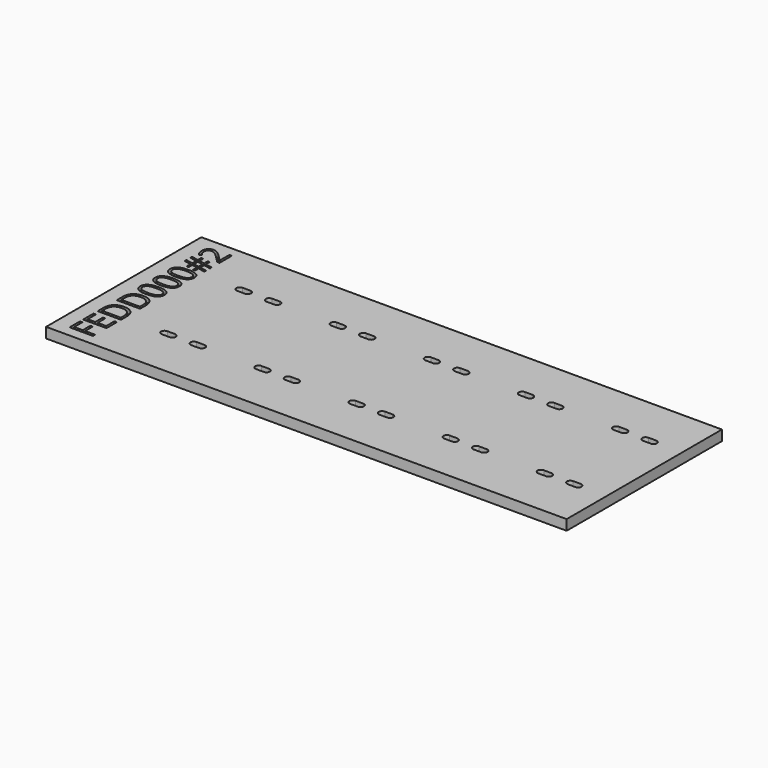
from build123d import *

# Parameters (mm, degrees)
F0_W         = 177
F0_H         = 66
F1_DEPTH     = 3.5
F2_TEXT_SIZE = 11.1111111111
F3_DEPTH     = 1.5
F5_DEPTH     = 3.5
F6_T1_DEPTH  = 3.5


# Not quite as in the source:
# - a fillet or chamfer that OpenCascade refuses, or shapes differently, is made with other operations: its cross-section is extruded or revolved along the edge and cut away or added
# - Text() gives the source's letters only with a copy of the font that has no kerning and outlines rounded to 1/6400 em; it was checked with that copy


with BuildPart() as f1:
    # F0 (on Top) → F1 (new body)
    with BuildSketch(Plane.XY):
        with Locations((0.9526101351, -16.284535466)):
            Rectangle(F0_W, F0_H)
    extrude(amount=F1_DEPTH)

    # F2 (on face) → F3 (cut)
    with BuildSketch(Plane.XY.offset(3.5)):
        with Locations(Location((-74.5473898649, -46.697535466), (0, 0, 90))):
            Text('FEDD000#2', F2_TEXT_SIZE, font='Open Sans', text_align=(TextAlign.LEFT, TextAlign.BOTTOM))
    extrude(amount=-F3_DEPTH, mode=Mode.SUBTRACT)

    # F4 (on face) → F5 (cut, through all)
    with BuildSketch(Plane.XY.offset(3.5)):
        with BuildLine():
            ThreePointArc((-59.5473898649, -1.434535466), (-58.7342170666, -1.0977082644), (-58.3973898649, -0.284535466))
            ThreePointArc((-58.3973898649, -0.284535466), (-58.7342170666, 0.5286373324), (-59.5473898649, 0.865464534))
            ThreePointArc((-59.5473898649, 0.865464534), (-60.6973898649, -0.284535466), (-59.5473898649, -1.434535466))
        make_face()
        with BuildLine():
            ThreePointArc((-59.5473898649, 0.865464534), (-58.7342170666, 0.5286373324), (-58.3973898649, -0.284535466))
            ThreePointArc((-58.3973898649, -0.284535466), (-58.7342170666, -1.0977082644), (-59.5473898649, -1.434535466))
            Line((-59.5473898649, -1.434535466), (-57.0473898649, -1.434535466))
            Line((-57.0473898649, -1.434535466), (-57.0473898649, 0.865464534))
            Line((-57.0473898649, 0.865464534), (-59.5473898649, 0.865464534))
        make_face()
        with BuildLine():
            ThreePointArc((-59.5473898649, -1.434535466), (-60.6973898649, -0.284535466), (-59.5473898649, 0.865464534))
            Line((-59.5473898649, 0.865464534), (-62.0473898649, 0.865464534))
            Line((-62.0473898649, 0.865464534), (-62.0473898649, -1.434535466))
            Line((-62.0473898649, -1.434535466), (-59.5473898649, -1.434535466))
        make_face()
        with BuildLine():
            ThreePointArc((-49.5473898649, -1.434535466), (-48.7342170666, -1.0977082644), (-48.3973898649, -0.284535466))
            ThreePointArc((-48.3973898649, -0.284535466), (-48.7342170666, 0.5286373324), (-49.5473898649, 0.865464534))
            ThreePointArc((-49.5473898649, 0.865464534), (-50.6973898649, -0.284535466), (-49.5473898649, -1.434535466))
        make_face()
        with BuildLine():
            ThreePointArc((-49.5473898649, 0.865464534), (-48.7342170666, 0.5286373324), (-48.3973898649, -0.284535466))
            ThreePointArc((-48.3973898649, -0.284535466), (-48.7342170666, -1.0977082644), (-49.5473898649, -1.434535466))
            Line((-49.5473898649, -1.434535466), (-47.0473898649, -1.434535466))
            Line((-47.0473898649, -1.434535466), (-47.0473898649, 0.865464534))
            Line((-47.0473898649, 0.865464534), (-49.5473898649, 0.865464534))
        make_face()
        with BuildLine():
            ThreePointArc((-49.5473898649, -1.434535466), (-50.6973898649, -0.284535466), (-49.5473898649, 0.865464534))
            Line((-49.5473898649, 0.865464534), (-52.0473898649, 0.865464534))
            Line((-52.0473898649, 0.865464534), (-52.0473898649, -1.434535466))
            Line((-52.0473898649, -1.434535466), (-49.5473898649, -1.434535466))
        make_face()
        with BuildLine():
            ThreePointArc((-27.5473898649, -1.434535466), (-26.7342170666, -1.0977082644), (-26.3973898649, -0.284535466))
            ThreePointArc((-26.3973898649, -0.284535466), (-26.7342170666, 0.5286373324), (-27.5473898649, 0.865464534))
            ThreePointArc((-27.5473898649, 0.865464534), (-28.6973898649, -0.284535466), (-27.5473898649, -1.434535466))
        make_face()
        with BuildLine():
            ThreePointArc((-27.5473898649, 0.865464534), (-26.7342170666, 0.5286373324), (-26.3973898649, -0.284535466))
            ThreePointArc((-26.3973898649, -0.284535466), (-26.7342170666, -1.0977082644), (-27.5473898649, -1.434535466))
            Line((-27.5473898649, -1.434535466), (-25.0473898649, -1.434535466))
            Line((-25.0473898649, -1.434535466), (-25.0473898649, 0.865464534))
            Line((-25.0473898649, 0.865464534), (-27.5473898649, 0.865464534))
        make_face()
        with BuildLine():
            ThreePointArc((-27.5473898649, -1.434535466), (-28.6973898649, -0.284535466), (-27.5473898649, 0.865464534))
            Line((-27.5473898649, 0.865464534), (-30.0473898649, 0.865464534))
            Line((-30.0473898649, 0.865464534), (-30.0473898649, -1.434535466))
            Line((-30.0473898649, -1.434535466), (-27.5473898649, -1.434535466))
        make_face()
        with BuildLine():
            ThreePointArc((-17.5473898649, -1.434535466), (-16.7342170666, -1.0977082644), (-16.3973898649, -0.284535466))
            ThreePointArc((-16.3973898649, -0.284535466), (-16.7342170666, 0.5286373324), (-17.5473898649, 0.865464534))
            ThreePointArc((-17.5473898649, 0.865464534), (-18.6973898649, -0.284535466), (-17.5473898649, -1.434535466))
        make_face()
        with BuildLine():
            ThreePointArc((-17.5473898649, 0.865464534), (-16.7342170666, 0.5286373324), (-16.3973898649, -0.284535466))
            ThreePointArc((-16.3973898649, -0.284535466), (-16.7342170666, -1.0977082644), (-17.5473898649, -1.434535466))
            Line((-17.5473898649, -1.434535466), (-15.0473898649, -1.434535466))
            Line((-15.0473898649, -1.434535466), (-15.0473898649, 0.865464534))
            Line((-15.0473898649, 0.865464534), (-17.5473898649, 0.865464534))
        make_face()
        with BuildLine():
            ThreePointArc((-17.5473898649, -1.434535466), (-18.6973898649, -0.284535466), (-17.5473898649, 0.865464534))
            Line((-17.5473898649, 0.865464534), (-20.0473898649, 0.865464534))
            Line((-20.0473898649, 0.865464534), (-20.0473898649, -1.434535466))
            Line((-20.0473898649, -1.434535466), (-17.5473898649, -1.434535466))
        make_face()
        with BuildLine():
            ThreePointArc((4.4526101351, -1.434535466), (5.2657829334, -1.0977082644), (5.6026101351, -0.284535466))
            ThreePointArc((5.6026101351, -0.284535466), (5.2657829334, 0.5286373324), (4.4526101351, 0.865464534))
            ThreePointArc((4.4526101351, 0.865464534), (3.3026101351, -0.284535466), (4.4526101351, -1.434535466))
        make_face()
        with BuildLine():
            ThreePointArc((4.4526101351, 0.865464534), (5.2657829334, 0.5286373324), (5.6026101351, -0.284535466))
            ThreePointArc((5.6026101351, -0.284535466), (5.2657829334, -1.0977082644), (4.4526101351, -1.434535466))
            Line((4.4526101351, -1.434535466), (6.9526101351, -1.434535466))
            Line((6.9526101351, -1.434535466), (6.9526101351, 0.865464534))
            Line((6.9526101351, 0.865464534), (4.4526101351, 0.865464534))
        make_face()
        with BuildLine():
            ThreePointArc((4.4526101351, -1.434535466), (3.3026101351, -0.284535466), (4.4526101351, 0.865464534))
            Line((4.4526101351, 0.865464534), (1.9526101351, 0.865464534))
            Line((1.9526101351, 0.865464534), (1.9526101351, -1.434535466))
            Line((1.9526101351, -1.434535466), (4.4526101351, -1.434535466))
        make_face()
        with BuildLine():
            ThreePointArc((14.4526101316, -1.434535466), (15.2657829322, -1.0977082656), (15.6026101351, -0.284535466))
            ThreePointArc((15.6026101351, -0.284535466), (15.2657829334, 0.5286373324), (14.4526101351, 0.865464534))
            ThreePointArc((14.4526101351, 0.865464534), (13.3026101351, -0.2845354643), (14.4526101316, -1.434535466))
        make_face()
        with BuildLine():
            ThreePointArc((14.4526101351, 0.865464534), (15.2657829334, 0.5286373324), (15.6026101351, -0.284535466))
            ThreePointArc((15.6026101351, -0.284535466), (15.2657829322, -1.0977082656), (14.4526101316, -1.434535466))
            Line((14.4526101316, -1.434535466), (16.9526101351, -1.434535466))
            Line((16.9526101351, -1.434535466), (16.9526101351, 0.865464534))
            Line((16.9526101351, 0.865464534), (14.4526101351, 0.865464534))
        make_face()
        with BuildLine():
            ThreePointArc((14.4526101316, -1.434535466), (13.3026101351, -0.2845354643), (14.4526101351, 0.865464534))
            Line((14.4526101351, 0.865464534), (11.9526101351, 0.865464534))
            Line((11.9526101351, 0.865464534), (11.9526101351, -1.434535466))
            Line((11.9526101351, -1.434535466), (14.4526101316, -1.434535466))
        make_face()
        with BuildLine():
            ThreePointArc((36.4526101351, -1.434535466), (37.2657829334, -1.0977082644), (37.6026101351, -0.284535466))
            ThreePointArc((37.6026101351, -0.284535466), (37.2657829334, 0.5286373324), (36.4526101351, 0.865464534))
            ThreePointArc((36.4526101351, 0.865464534), (35.3026101351, -0.284535466), (36.4526101351, -1.434535466))
        make_face()
        with BuildLine():
            ThreePointArc((36.4526101351, 0.865464534), (37.2657829334, 0.5286373324), (37.6026101351, -0.284535466))
            ThreePointArc((37.6026101351, -0.284535466), (37.2657829334, -1.0977082644), (36.4526101351, -1.434535466))
            Line((36.4526101351, -1.434535466), (38.9526101351, -1.434535466))
            Line((38.9526101351, -1.434535466), (38.9526101351, 0.865464534))
            Line((38.9526101351, 0.865464534), (36.4526101351, 0.865464534))
        make_face()
        with BuildLine():
            ThreePointArc((36.4526101351, -1.434535466), (35.3026101351, -0.284535466), (36.4526101351, 0.865464534))
            Line((36.4526101351, 0.865464534), (33.9526101351, 0.865464534))
            Line((33.9526101351, 0.865464534), (33.9526101351, -1.434535466))
            Line((33.9526101351, -1.434535466), (36.4526101351, -1.434535466))
        make_face()
        with BuildLine():
            ThreePointArc((46.4526101351, -1.434535466), (47.2657829334, -1.0977082644), (47.6026101351, -0.284535466))
            ThreePointArc((47.6026101351, -0.284535466), (47.2657829334, 0.5286373324), (46.4526101351, 0.865464534))
            ThreePointArc((46.4526101351, 0.865464534), (45.3026101351, -0.284535466), (46.4526101351, -1.434535466))
        make_face()
        with BuildLine():
            ThreePointArc((46.4526101351, 0.865464534), (47.2657829334, 0.5286373324), (47.6026101351, -0.284535466))
            ThreePointArc((47.6026101351, -0.284535466), (47.2657829334, -1.0977082644), (46.4526101351, -1.434535466))
            Line((46.4526101351, -1.434535466), (48.9526101351, -1.434535466))
            Line((48.9526101351, -1.434535466), (48.9526101351, 0.865464534))
            Line((48.9526101351, 0.865464534), (46.4526101351, 0.865464534))
        make_face()
        with BuildLine():
            ThreePointArc((46.4526101351, -1.434535466), (45.3026101351, -0.284535466), (46.4526101351, 0.865464534))
            Line((46.4526101351, 0.865464534), (43.9526101351, 0.865464534))
            Line((43.9526101351, 0.865464534), (43.9526101351, -1.434535466))
            Line((43.9526101351, -1.434535466), (46.4526101351, -1.434535466))
        make_face()
        with BuildLine():
            ThreePointArc((68.4526101316, -1.434535466), (69.2657829322, -1.0977082656), (69.6026101351, -0.284535466))
            ThreePointArc((69.6026101351, -0.284535466), (69.2657829334, 0.5286373324), (68.4526101351, 0.865464534))
            ThreePointArc((68.4526101351, 0.865464534), (67.3026101351, -0.2845354643), (68.4526101316, -1.434535466))
        make_face()
        with BuildLine():
            ThreePointArc((68.4526101351, 0.865464534), (69.2657829334, 0.5286373324), (69.6026101351, -0.284535466))
            ThreePointArc((69.6026101351, -0.284535466), (69.2657829322, -1.0977082656), (68.4526101316, -1.434535466))
            Line((68.4526101316, -1.434535466), (70.9526101351, -1.434535466))
            Line((70.9526101351, -1.434535466), (70.9526101351, 0.865464534))
            Line((70.9526101351, 0.865464534), (68.4526101351, 0.865464534))
        make_face()
        with BuildLine():
            ThreePointArc((68.4526101316, -1.434535466), (67.3026101351, -0.2845354643), (68.4526101351, 0.865464534))
            Line((68.4526101351, 0.865464534), (65.9526101351, 0.865464534))
            Line((65.9526101351, 0.865464534), (65.9526101351, -1.434535466))
            Line((65.9526101351, -1.434535466), (68.4526101316, -1.434535466))
        make_face()
        with BuildLine():
            ThreePointArc((78.4526101351, -1.434535466), (79.2657829334, -1.0977082644), (79.6026101351, -0.284535466))
            ThreePointArc((79.6026101351, -0.284535466), (79.2657829334, 0.5286373324), (78.4526101351, 0.865464534))
            ThreePointArc((78.4526101351, 0.865464534), (77.3026101351, -0.284535466), (78.4526101351, -1.434535466))
        make_face()
        with BuildLine():
            ThreePointArc((78.4526101351, 0.865464534), (79.2657829334, 0.5286373324), (79.6026101351, -0.284535466))
            ThreePointArc((79.6026101351, -0.284535466), (79.2657829334, -1.0977082644), (78.4526101351, -1.434535466))
            Line((78.4526101351, -1.434535466), (80.9526101351, -1.434535466))
            Line((80.9526101351, -1.434535466), (80.9526101351, 0.865464534))
            Line((80.9526101351, 0.865464534), (78.4526101351, 0.865464534))
        make_face()
        with BuildLine():
            ThreePointArc((78.4526101351, -1.434535466), (77.3026101351, -0.284535466), (78.4526101351, 0.865464534))
            Line((78.4526101351, 0.865464534), (75.9526101351, 0.865464534))
            Line((75.9526101351, 0.865464534), (75.9526101351, -1.434535466))
            Line((75.9526101351, -1.434535466), (78.4526101351, -1.434535466))
        make_face()
        with BuildLine():
            ThreePointArc((-59.5473898649, -33.434535466), (-58.7342170666, -33.0977082644), (-58.3973898649, -32.284535466))
            ThreePointArc((-58.3973898649, -32.284535466), (-58.7342170666, -31.4713626676), (-59.5473898649, -31.134535466))
            ThreePointArc((-59.5473898649, -31.134535466), (-60.6973898649, -32.284535466), (-59.5473898649, -33.434535466))
        make_face()
        with BuildLine():
            ThreePointArc((-59.5473898649, -31.134535466), (-58.7342170666, -31.4713626676), (-58.3973898649, -32.284535466))
            ThreePointArc((-58.3973898649, -32.284535466), (-58.7342170666, -33.0977082644), (-59.5473898649, -33.434535466))
            Line((-59.5473898649, -33.434535466), (-57.0473898649, -33.434535466))
            Line((-57.0473898649, -33.434535466), (-57.0473898649, -31.134535466))
            Line((-57.0473898649, -31.134535466), (-59.5473898649, -31.134535466))
        make_face()
        with BuildLine():
            ThreePointArc((-59.5473898649, -33.434535466), (-60.6973898649, -32.284535466), (-59.5473898649, -31.134535466))
            Line((-59.5473898649, -31.134535466), (-62.0473898649, -31.134535466))
            Line((-62.0473898649, -31.134535466), (-62.0473898649, -33.434535466))
            Line((-62.0473898649, -33.434535466), (-59.5473898649, -33.434535466))
        make_face()
        with BuildLine():
            ThreePointArc((-49.5473898649, -33.434535466), (-48.7342170666, -33.0977082644), (-48.3973898649, -32.284535466))
            ThreePointArc((-48.3973898649, -32.284535466), (-48.7342170666, -31.4713626676), (-49.5473898649, -31.134535466))
            ThreePointArc((-49.5473898649, -31.134535466), (-50.6973898649, -32.284535466), (-49.5473898649, -33.434535466))
        make_face()
        with BuildLine():
            ThreePointArc((-49.5473898649, -31.134535466), (-48.7342170666, -31.4713626676), (-48.3973898649, -32.284535466))
            ThreePointArc((-48.3973898649, -32.284535466), (-48.7342170666, -33.0977082644), (-49.5473898649, -33.434535466))
            Line((-49.5473898649, -33.434535466), (-47.0473898649, -33.434535466))
            Line((-47.0473898649, -33.434535466), (-47.0473898649, -31.134535466))
            Line((-47.0473898649, -31.134535466), (-49.5473898649, -31.134535466))
        make_face()
        with BuildLine():
            ThreePointArc((-49.5473898649, -33.434535466), (-50.6973898649, -32.284535466), (-49.5473898649, -31.134535466))
            Line((-49.5473898649, -31.134535466), (-52.0473898649, -31.134535466))
            Line((-52.0473898649, -31.134535466), (-52.0473898649, -33.434535466))
            Line((-52.0473898649, -33.434535466), (-49.5473898649, -33.434535466))
        make_face()
        with BuildLine():
            ThreePointArc((-27.5473898649, -33.434535466), (-26.7342170666, -33.0977082644), (-26.3973898649, -32.284535466))
            ThreePointArc((-26.3973898649, -32.284535466), (-26.7342170666, -31.4713626676), (-27.5473898649, -31.134535466))
            ThreePointArc((-27.5473898649, -31.134535466), (-28.6973898649, -32.284535466), (-27.5473898649, -33.434535466))
        make_face()
        with BuildLine():
            ThreePointArc((-27.5473898649, -31.134535466), (-26.7342170666, -31.4713626676), (-26.3973898649, -32.284535466))
            ThreePointArc((-26.3973898649, -32.284535466), (-26.7342170666, -33.0977082644), (-27.5473898649, -33.434535466))
            Line((-27.5473898649, -33.434535466), (-25.0473898649, -33.434535466))
            Line((-25.0473898649, -33.434535466), (-25.0473898649, -31.134535466))
            Line((-25.0473898649, -31.134535466), (-27.5473898649, -31.134535466))
        make_face()
        with BuildLine():
            ThreePointArc((-27.5473898649, -33.434535466), (-28.6973898649, -32.284535466), (-27.5473898649, -31.134535466))
            Line((-27.5473898649, -31.134535466), (-30.0473898649, -31.134535466))
            Line((-30.0473898649, -31.134535466), (-30.0473898649, -33.434535466))
            Line((-30.0473898649, -33.434535466), (-27.5473898649, -33.434535466))
        make_face()
        with BuildLine():
            ThreePointArc((-17.5473898649, -33.434535466), (-16.7342170666, -33.0977082644), (-16.3973898649, -32.284535466))
            ThreePointArc((-16.3973898649, -32.284535466), (-16.7342170666, -31.4713626676), (-17.5473898649, -31.134535466))
            ThreePointArc((-17.5473898649, -31.134535466), (-18.6973898649, -32.284535466), (-17.5473898649, -33.434535466))
        make_face()
        with BuildLine():
            ThreePointArc((-17.5473898649, -31.134535466), (-16.7342170666, -31.4713626676), (-16.3973898649, -32.284535466))
            ThreePointArc((-16.3973898649, -32.284535466), (-16.7342170666, -33.0977082644), (-17.5473898649, -33.434535466))
            Line((-17.5473898649, -33.434535466), (-15.0473898649, -33.434535466))
            Line((-15.0473898649, -33.434535466), (-15.0473898649, -31.134535466))
            Line((-15.0473898649, -31.134535466), (-17.5473898649, -31.134535466))
        make_face()
        with BuildLine():
            ThreePointArc((-17.5473898649, -33.434535466), (-18.6973898649, -32.284535466), (-17.5473898649, -31.134535466))
            Line((-17.5473898649, -31.134535466), (-20.0473898649, -31.134535466))
            Line((-20.0473898649, -31.134535466), (-20.0473898649, -33.434535466))
            Line((-20.0473898649, -33.434535466), (-17.5473898649, -33.434535466))
        make_face()
        with BuildLine():
            ThreePointArc((4.4526101351, -33.434535466), (5.2657829334, -33.0977082644), (5.6026101351, -32.284535466))
            ThreePointArc((5.6026101351, -32.284535466), (5.2657829334, -31.4713626676), (4.4526101351, -31.134535466))
            ThreePointArc((4.4526101351, -31.134535466), (3.3026101351, -32.284535466), (4.4526101351, -33.434535466))
        make_face()
        with BuildLine():
            ThreePointArc((4.4526101351, -31.134535466), (5.2657829334, -31.4713626676), (5.6026101351, -32.284535466))
            ThreePointArc((5.6026101351, -32.284535466), (5.2657829334, -33.0977082644), (4.4526101351, -33.434535466))
            Line((4.4526101351, -33.434535466), (6.9526101351, -33.434535466))
            Line((6.9526101351, -33.434535466), (6.9526101351, -31.134535466))
            Line((6.9526101351, -31.134535466), (4.4526101351, -31.134535466))
        make_face()
        with BuildLine():
            ThreePointArc((4.4526101351, -33.434535466), (3.3026101351, -32.284535466), (4.4526101351, -31.134535466))
            Line((4.4526101351, -31.134535466), (1.9526101351, -31.134535466))
            Line((1.9526101351, -31.134535466), (1.9526101351, -33.434535466))
            Line((1.9526101351, -33.434535466), (4.4526101351, -33.434535466))
        make_face()
        with BuildLine():
            ThreePointArc((14.4526101351, -33.434535466), (15.2657829334, -33.0977082644), (15.6026101351, -32.284535466))
            ThreePointArc((15.6026101351, -32.284535466), (15.2657829334, -31.4713626676), (14.4526101351, -31.134535466))
            ThreePointArc((14.4526101351, -31.134535466), (13.3026101351, -32.284535466), (14.4526101351, -33.434535466))
        make_face()
        with BuildLine():
            ThreePointArc((14.4526101351, -31.134535466), (15.2657829334, -31.4713626676), (15.6026101351, -32.284535466))
            ThreePointArc((15.6026101351, -32.284535466), (15.2657829334, -33.0977082644), (14.4526101351, -33.434535466))
            Line((14.4526101351, -33.434535466), (16.9526101351, -33.434535466))
            Line((16.9526101351, -33.434535466), (16.9526101351, -31.134535466))
            Line((16.9526101351, -31.134535466), (14.4526101351, -31.134535466))
        make_face()
        with BuildLine():
            ThreePointArc((14.4526101351, -33.434535466), (13.3026101351, -32.284535466), (14.4526101351, -31.134535466))
            Line((14.4526101351, -31.134535466), (11.9526101351, -31.134535466))
            Line((11.9526101351, -31.134535466), (11.9526101351, -33.434535466))
            Line((11.9526101351, -33.434535466), (14.4526101351, -33.434535466))
        make_face()
        with BuildLine():
            ThreePointArc((36.4526101351, -33.434535466), (37.2657829334, -33.0977082644), (37.6026101351, -32.284535466))
            ThreePointArc((37.6026101351, -32.284535466), (37.2657829334, -31.4713626676), (36.4526101351, -31.134535466))
            ThreePointArc((36.4526101351, -31.134535466), (35.3026101351, -32.284535466), (36.4526101351, -33.434535466))
        make_face()
        with BuildLine():
            ThreePointArc((36.4526101351, -31.134535466), (37.2657829334, -31.4713626676), (37.6026101351, -32.284535466))
            ThreePointArc((37.6026101351, -32.284535466), (37.2657829334, -33.0977082644), (36.4526101351, -33.434535466))
            Line((36.4526101351, -33.434535466), (38.9526101351, -33.434535466))
            Line((38.9526101351, -33.434535466), (38.9526101351, -31.134535466))
            Line((38.9526101351, -31.134535466), (36.4526101351, -31.134535466))
        make_face()
        with BuildLine():
            ThreePointArc((36.4526101351, -33.434535466), (35.3026101351, -32.284535466), (36.4526101351, -31.134535466))
            Line((36.4526101351, -31.134535466), (33.9526101351, -31.134535466))
            Line((33.9526101351, -31.134535466), (33.9526101351, -33.434535466))
            Line((33.9526101351, -33.434535466), (36.4526101351, -33.434535466))
        make_face()
        with BuildLine():
            ThreePointArc((46.4526101351, -33.434535466), (47.2657829334, -33.0977082644), (47.6026101351, -32.284535466))
            ThreePointArc((47.6026101351, -32.284535466), (47.2657829334, -31.4713626676), (46.4526101351, -31.134535466))
            ThreePointArc((46.4526101351, -31.134535466), (45.3026101351, -32.284535466), (46.4526101351, -33.434535466))
        make_face()
        with BuildLine():
            ThreePointArc((46.4526101351, -31.134535466), (47.2657829334, -31.4713626676), (47.6026101351, -32.284535466))
            ThreePointArc((47.6026101351, -32.284535466), (47.2657829334, -33.0977082644), (46.4526101351, -33.434535466))
            Line((46.4526101351, -33.434535466), (48.9526101351, -33.434535466))
            Line((48.9526101351, -33.434535466), (48.9526101351, -31.134535466))
            Line((48.9526101351, -31.134535466), (46.4526101351, -31.134535466))
        make_face()
        with BuildLine():
            ThreePointArc((46.4526101351, -33.434535466), (45.3026101351, -32.284535466), (46.4526101351, -31.134535466))
            Line((46.4526101351, -31.134535466), (43.9526101351, -31.134535466))
            Line((43.9526101351, -31.134535466), (43.9526101351, -33.434535466))
            Line((43.9526101351, -33.434535466), (46.4526101351, -33.434535466))
        make_face()
        with BuildLine():
            ThreePointArc((68.4526101351, -33.434535466), (69.2657829334, -33.0977082644), (69.6026101351, -32.284535466))
            ThreePointArc((69.6026101351, -32.284535466), (69.2657829334, -31.4713626676), (68.4526101351, -31.134535466))
            ThreePointArc((68.4526101351, -31.134535466), (67.3026101351, -32.284535466), (68.4526101351, -33.434535466))
        make_face()
        with BuildLine():
            ThreePointArc((68.4526101351, -31.134535466), (69.2657829334, -31.4713626676), (69.6026101351, -32.284535466))
            ThreePointArc((69.6026101351, -32.284535466), (69.2657829334, -33.0977082644), (68.4526101351, -33.434535466))
            Line((68.4526101351, -33.434535466), (70.9526101351, -33.434535466))
            Line((70.9526101351, -33.434535466), (70.9526101351, -31.134535466))
            Line((70.9526101351, -31.134535466), (68.4526101351, -31.134535466))
        make_face()
        with BuildLine():
            ThreePointArc((68.4526101351, -33.434535466), (67.3026101351, -32.284535466), (68.4526101351, -31.134535466))
            Line((68.4526101351, -31.134535466), (65.9526101351, -31.134535466))
            Line((65.9526101351, -31.134535466), (65.9526101351, -33.434535466))
            Line((65.9526101351, -33.434535466), (68.4526101351, -33.434535466))
        make_face()
        with BuildLine():
            ThreePointArc((78.4526101351, -33.434535466), (79.2657829334, -33.0977082644), (79.6026101351, -32.284535466))
            ThreePointArc((79.6026101351, -32.284535466), (79.2657829334, -31.4713626676), (78.4526101351, -31.134535466))
            ThreePointArc((78.4526101351, -31.134535466), (77.3026101351, -32.284535466), (78.4526101351, -33.434535466))
        make_face()
        with BuildLine():
            ThreePointArc((78.4526101351, -31.134535466), (79.2657829334, -31.4713626676), (79.6026101351, -32.284535466))
            ThreePointArc((79.6026101351, -32.284535466), (79.2657829334, -33.0977082644), (78.4526101351, -33.434535466))
            Line((78.4526101351, -33.434535466), (80.9526101351, -33.434535466))
            Line((80.9526101351, -33.434535466), (80.9526101351, -31.134535466))
            Line((80.9526101351, -31.134535466), (78.4526101351, -31.134535466))
        make_face()
        with BuildLine():
            ThreePointArc((78.4526101351, -33.434535466), (77.3026101351, -32.284535466), (78.4526101351, -31.134535466))
            Line((78.4526101351, -31.134535466), (75.9526101351, -31.134535466))
            Line((75.9526101351, -31.134535466), (75.9526101351, -33.434535466))
            Line((75.9526101351, -33.434535466), (78.4526101351, -33.434535466))
        make_face()
    extrude(amount=-F5_DEPTH, mode=Mode.SUBTRACT)

    # F6: fillet of radius 1.2 on 80 edges, made by hand

    # F6_s2 → F6_t1 (join)
    with BuildSketch(Plane.XY):
        with BuildLine():
            ThreePointArc((-62.0473898649, -0.334535466), (-61.6959180023, 0.5139926714), (-60.8473898649, 0.865464534))
            Line((-60.8473898649, 0.865464534), (-62.0473898649, 0.865464534))
            Line((-62.0473898649, 0.865464534), (-62.0473898649, -0.334535466))
        make_face()
        with BuildLine():
            ThreePointArc((-50.8473898649, 0.865464534), (-51.6959180023, 0.5139926714), (-52.0473898649, -0.334535466))
            Line((-52.0473898649, -0.334535466), (-52.0473898649, 0.865464534))
            Line((-52.0473898649, 0.865464534), (-50.8473898649, 0.865464534))
        make_face()
        with BuildLine():
            ThreePointArc((-28.8473898649, 0.865464534), (-29.6959180023, 0.5139926714), (-30.0473898649, -0.334535466))
            Line((-30.0473898649, -0.334535466), (-30.0473898649, 0.865464534))
            Line((-30.0473898649, 0.865464534), (-28.8473898649, 0.865464534))
        make_face()
        with BuildLine():
            ThreePointArc((-18.8473898649, 0.865464534), (-19.6959180023, 0.5139926714), (-20.0473898649, -0.334535466))
            Line((-20.0473898649, -0.334535466), (-20.0473898649, 0.865464534))
            Line((-20.0473898649, 0.865464534), (-18.8473898649, 0.865464534))
        make_face()
        with BuildLine():
            ThreePointArc((3.1526101351, 0.865464534), (2.3040819977, 0.5139926714), (1.9526101351, -0.334535466))
            Line((1.9526101351, -0.334535466), (1.9526101351, 0.865464534))
            Line((1.9526101351, 0.865464534), (3.1526101351, 0.865464534))
        make_face()
        with BuildLine():
            ThreePointArc((13.1526101351, 0.865464534), (12.3040819977, 0.5139926714), (11.9526101351, -0.334535466))
            Line((11.9526101351, -0.334535466), (11.9526101351, 0.865464534))
            Line((11.9526101351, 0.865464534), (13.1526101351, 0.865464534))
        make_face()
        with BuildLine():
            ThreePointArc((35.1526101351, 0.865464534), (34.3040819977, 0.5139926714), (33.9526101351, -0.334535466))
            Line((33.9526101351, -0.334535466), (33.9526101351, 0.865464534))
            Line((33.9526101351, 0.865464534), (35.1526101351, 0.865464534))
        make_face()
        with BuildLine():
            ThreePointArc((43.9526101351, -0.334535466), (44.3040819977, 0.5139926714), (45.1526101351, 0.865464534))
            Line((45.1526101351, 0.865464534), (43.9526101351, 0.865464534))
            Line((43.9526101351, 0.865464534), (43.9526101351, -0.334535466))
        make_face()
        with BuildLine():
            ThreePointArc((67.1526101351, 0.865464534), (66.3040819977, 0.5139926714), (65.9526101351, -0.334535466))
            Line((65.9526101351, -0.334535466), (65.9526101351, 0.865464534))
            Line((65.9526101351, 0.865464534), (67.1526101351, 0.865464534))
        make_face()
        with BuildLine():
            ThreePointArc((77.1526101351, 0.865464534), (76.3040819977, 0.5139926714), (75.9526101351, -0.334535466))
            Line((75.9526101351, -0.334535466), (75.9526101351, 0.865464534))
            Line((75.9526101351, 0.865464534), (77.1526101351, 0.865464534))
        make_face()
        with BuildLine():
            ThreePointArc((77.1526101351, -31.134535466), (76.3040819977, -31.4860073286), (75.9526101351, -32.334535466))
            Line((75.9526101351, -32.334535466), (75.9526101351, -31.134535466))
            Line((75.9526101351, -31.134535466), (77.1526101351, -31.134535466))
        make_face()
        with BuildLine():
            ThreePointArc((67.1526101351, -31.134535466), (66.3040819977, -31.4860073286), (65.9526101351, -32.334535466))
            Line((65.9526101351, -32.334535466), (65.9526101351, -31.134535466))
            Line((65.9526101351, -31.134535466), (67.1526101351, -31.134535466))
        make_face()
        with BuildLine():
            ThreePointArc((45.1526101351, -31.134535466), (44.3040819977, -31.4860073286), (43.9526101351, -32.334535466))
            Line((43.9526101351, -32.334535466), (43.9526101351, -31.134535466))
            Line((43.9526101351, -31.134535466), (45.1526101351, -31.134535466))
        make_face()
        with BuildLine():
            ThreePointArc((-28.8473898649, -31.134535466), (-29.6959180023, -31.4860073286), (-30.0473898649, -32.334535466))
            Line((-30.0473898649, -32.334535466), (-30.0473898649, -31.134535466))
            Line((-30.0473898649, -31.134535466), (-28.8473898649, -31.134535466))
        make_face()
        with BuildLine():
            ThreePointArc((-18.8473898649, -31.134535466), (-19.6959180023, -31.4860073286), (-20.0473898649, -32.334535466))
            Line((-20.0473898649, -32.334535466), (-20.0473898649, -31.134535466))
            Line((-20.0473898649, -31.134535466), (-18.8473898649, -31.134535466))
        make_face()
        with BuildLine():
            ThreePointArc((3.1526101351, -31.134535466), (2.3040819977, -31.4860073286), (1.9526101351, -32.334535466))
            Line((1.9526101351, -32.334535466), (1.9526101351, -31.134535466))
            Line((1.9526101351, -31.134535466), (3.1526101351, -31.134535466))
        make_face()
        with BuildLine():
            ThreePointArc((13.1526101351, -31.134535466), (12.3040819977, -31.4860073286), (11.9526101351, -32.334535466))
            Line((11.9526101351, -32.334535466), (11.9526101351, -31.134535466))
            Line((11.9526101351, -31.134535466), (13.1526101351, -31.134535466))
        make_face()
        with BuildLine():
            ThreePointArc((35.1526101351, -31.134535466), (34.3040819977, -31.4860073286), (33.9526101351, -32.334535466))
            Line((33.9526101351, -32.334535466), (33.9526101351, -31.134535466))
            Line((33.9526101351, -31.134535466), (35.1526101351, -31.134535466))
        make_face()
        with BuildLine():
            ThreePointArc((-60.8473898649, -31.134535466), (-61.6959180023, -31.4860073286), (-62.0473898649, -32.334535466))
            Line((-62.0473898649, -32.334535466), (-62.0473898649, -31.134535466))
            Line((-62.0473898649, -31.134535466), (-60.8473898649, -31.134535466))
        make_face()
        with BuildLine():
            ThreePointArc((-50.8473898649, -31.134535466), (-51.6959180023, -31.4860073286), (-52.0473898649, -32.334535466))
            Line((-52.0473898649, -32.334535466), (-52.0473898649, -31.134535466))
            Line((-52.0473898649, -31.134535466), (-50.8473898649, -31.134535466))
        make_face()
        with BuildLine():
            ThreePointArc((-57.0473898649, -0.334535466), (-57.3988617275, 0.5139926714), (-58.2473898649, 0.865464534))
            Line((-58.2473898649, 0.865464534), (-57.0473898649, 0.865464534))
            Line((-57.0473898649, 0.865464534), (-57.0473898649, -0.334535466))
        make_face()
        with BuildLine():
            ThreePointArc((-47.0473898649, -0.334535466), (-47.3988617275, 0.5139926714), (-48.2473898649, 0.865464534))
            Line((-48.2473898649, 0.865464534), (-47.0473898649, 0.865464534))
            Line((-47.0473898649, 0.865464534), (-47.0473898649, -0.334535466))
        make_face()
        with BuildLine():
            ThreePointArc((-25.0473898649, -0.334535466), (-25.3988617275, 0.5139926714), (-26.2473898649, 0.865464534))
            Line((-26.2473898649, 0.865464534), (-25.0473898649, 0.865464534))
            Line((-25.0473898649, 0.865464534), (-25.0473898649, -0.334535466))
        make_face()
        with BuildLine():
            ThreePointArc((-15.0473898649, -0.334535466), (-15.3988617275, 0.5139926714), (-16.2473898649, 0.865464534))
            Line((-16.2473898649, 0.865464534), (-15.0473898649, 0.865464534))
            Line((-15.0473898649, 0.865464534), (-15.0473898649, -0.334535466))
        make_face()
        with BuildLine():
            ThreePointArc((6.9526101351, -0.334535466), (6.6011382725, 0.5139926714), (5.7526101351, 0.865464534))
            Line((5.7526101351, 0.865464534), (6.9526101351, 0.865464534))
            Line((6.9526101351, 0.865464534), (6.9526101351, -0.334535466))
        make_face()
        with BuildLine():
            ThreePointArc((16.9526101351, -0.334535466), (16.6011382725, 0.5139926714), (15.7526101351, 0.865464534))
            Line((15.7526101351, 0.865464534), (16.9526101351, 0.865464534))
            Line((16.9526101351, 0.865464534), (16.9526101351, -0.334535466))
        make_face()
        with BuildLine():
            ThreePointArc((38.9526101351, -0.334535466), (38.6011382725, 0.5139926714), (37.7526101351, 0.865464534))
            Line((37.7526101351, 0.865464534), (38.9526101351, 0.865464534))
            Line((38.9526101351, 0.865464534), (38.9526101351, -0.334535466))
        make_face()
        with BuildLine():
            ThreePointArc((48.9526101351, -0.334535466), (48.6011382725, 0.5139926714), (47.7526101351, 0.865464534))
            Line((47.7526101351, 0.865464534), (48.9526101351, 0.865464534))
            Line((48.9526101351, 0.865464534), (48.9526101351, -0.334535466))
        make_face()
        with BuildLine():
            ThreePointArc((70.9526101351, -0.334535466), (70.6011382725, 0.5139926714), (69.7526101351, 0.865464534))
            Line((69.7526101351, 0.865464534), (70.9526101351, 0.865464534))
            Line((70.9526101351, 0.865464534), (70.9526101351, -0.334535466))
        make_face()
        with BuildLine():
            ThreePointArc((80.9526101351, -0.334535466), (80.6011382725, 0.5139926714), (79.7526101351, 0.865464534))
            Line((79.7526101351, 0.865464534), (80.9526101351, 0.865464534))
            Line((80.9526101351, 0.865464534), (80.9526101351, -0.334535466))
        make_face()
        with BuildLine():
            ThreePointArc((80.9526101351, -32.334535466), (80.6011382725, -31.4860073286), (79.7526101351, -31.134535466))
            Line((79.7526101351, -31.134535466), (80.9526101351, -31.134535466))
            Line((80.9526101351, -31.134535466), (80.9526101351, -32.334535466))
        make_face()
        with BuildLine():
            ThreePointArc((70.9526101351, -32.334535466), (70.6011382725, -31.4860073286), (69.7526101351, -31.134535466))
            Line((69.7526101351, -31.134535466), (70.9526101351, -31.134535466))
            Line((70.9526101351, -31.134535466), (70.9526101351, -32.334535466))
        make_face()
        with BuildLine():
            ThreePointArc((48.9526101351, -32.334535466), (48.6011382725, -31.4860073286), (47.7526101351, -31.134535466))
            Line((47.7526101351, -31.134535466), (48.9526101351, -31.134535466))
            Line((48.9526101351, -31.134535466), (48.9526101351, -32.334535466))
        make_face()
        with BuildLine():
            ThreePointArc((38.9526101351, -32.334535466), (38.6011382725, -31.4860073286), (37.7526101351, -31.134535466))
            Line((37.7526101351, -31.134535466), (38.9526101351, -31.134535466))
            Line((38.9526101351, -31.134535466), (38.9526101351, -32.334535466))
        make_face()
        with BuildLine():
            ThreePointArc((16.9526101351, -32.334535466), (16.6011382725, -31.4860073286), (15.7526101351, -31.134535466))
            Line((15.7526101351, -31.134535466), (16.9526101351, -31.134535466))
            Line((16.9526101351, -31.134535466), (16.9526101351, -32.334535466))
        make_face()
        with BuildLine():
            ThreePointArc((6.9526101351, -32.334535466), (6.6011382725, -31.4860073286), (5.7526101351, -31.134535466))
            Line((5.7526101351, -31.134535466), (6.9526101351, -31.134535466))
            Line((6.9526101351, -31.134535466), (6.9526101351, -32.334535466))
        make_face()
        with BuildLine():
            ThreePointArc((-15.0473898649, -32.334535466), (-15.3988617275, -31.4860073286), (-16.2473898649, -31.134535466))
            Line((-16.2473898649, -31.134535466), (-15.0473898649, -31.134535466))
            Line((-15.0473898649, -31.134535466), (-15.0473898649, -32.334535466))
        make_face()
        with BuildLine():
            ThreePointArc((-25.0473898649, -32.334535466), (-25.3988617275, -31.4860073286), (-26.2473898649, -31.134535466))
            Line((-26.2473898649, -31.134535466), (-25.0473898649, -31.134535466))
            Line((-25.0473898649, -31.134535466), (-25.0473898649, -32.334535466))
        make_face()
        with BuildLine():
            ThreePointArc((-47.0473898649, -32.334535466), (-47.3988617275, -31.4860073286), (-48.2473898649, -31.134535466))
            Line((-48.2473898649, -31.134535466), (-47.0473898649, -31.134535466))
            Line((-47.0473898649, -31.134535466), (-47.0473898649, -32.334535466))
        make_face()
        with BuildLine():
            ThreePointArc((-57.0473898649, -32.334535466), (-57.3988617275, -31.4860073286), (-58.2473898649, -31.134535466))
            Line((-58.2473898649, -31.134535466), (-57.0473898649, -31.134535466))
            Line((-57.0473898649, -31.134535466), (-57.0473898649, -32.334535466))
        make_face()
        with BuildLine():
            ThreePointArc((80.9526101351, -0.234535466), (80.6011382725, -1.0830636034), (79.7526101351, -1.434535466))
            Line((79.7526101351, -1.434535466), (80.9526101351, -1.434535466))
            Line((80.9526101351, -1.434535466), (80.9526101351, -0.234535466))
        make_face()
        with BuildLine():
            ThreePointArc((79.7526101351, -33.434535466), (80.6011382725, -33.0830636034), (80.9526101351, -32.234535466))
            Line((80.9526101351, -32.234535466), (80.9526101351, -33.434535466))
            Line((80.9526101351, -33.434535466), (79.7526101351, -33.434535466))
        make_face()
        with BuildLine():
            ThreePointArc((69.7526101351, -1.434535466), (70.6011382725, -1.0830636034), (70.9526101351, -0.234535466))
            Line((70.9526101351, -0.234535466), (70.9526101351, -1.434535466))
            Line((70.9526101351, -1.434535466), (69.7526101351, -1.434535466))
        make_face()
        with BuildLine():
            ThreePointArc((47.7526101351, -1.434535466), (48.6011382725, -1.0830636034), (48.9526101351, -0.234535466))
            Line((48.9526101351, -0.234535466), (48.9526101351, -1.434535466))
            Line((48.9526101351, -1.434535466), (47.7526101351, -1.434535466))
        make_face()
        with BuildLine():
            ThreePointArc((48.9526101351, -32.234535466), (48.6011382725, -33.0830636034), (47.7526101351, -33.434535466))
            Line((47.7526101351, -33.434535466), (48.9526101351, -33.434535466))
            Line((48.9526101351, -33.434535466), (48.9526101351, -32.234535466))
        make_face()
        with BuildLine():
            ThreePointArc((38.9526101351, -32.234535466), (38.6011382725, -33.0830636034), (37.7526101351, -33.434535466))
            Line((37.7526101351, -33.434535466), (38.9526101351, -33.434535466))
            Line((38.9526101351, -33.434535466), (38.9526101351, -32.234535466))
        make_face()
        with BuildLine():
            ThreePointArc((38.9526101351, -0.234535466), (38.6011382725, -1.0830636034), (37.7526101351, -1.434535466))
            Line((37.7526101351, -1.434535466), (38.9526101351, -1.434535466))
            Line((38.9526101351, -1.434535466), (38.9526101351, -0.234535466))
        make_face()
        with BuildLine():
            ThreePointArc((16.9526101351, -0.234535466), (16.6011382725, -1.0830636034), (15.7526101351, -1.434535466))
            Line((15.7526101351, -1.434535466), (16.9526101351, -1.434535466))
            Line((16.9526101351, -1.434535466), (16.9526101351, -0.234535466))
        make_face()
        with BuildLine():
            ThreePointArc((6.9526101351, -0.234535466), (6.6011382725, -1.0830636034), (5.7526101351, -1.434535466))
            Line((5.7526101351, -1.434535466), (6.9526101351, -1.434535466))
            Line((6.9526101351, -1.434535466), (6.9526101351, -0.234535466))
        make_face()
        with BuildLine():
            ThreePointArc((-16.2473898649, -1.434535466), (-15.3988617275, -1.0830636034), (-15.0473898649, -0.234535466))
            Line((-15.0473898649, -0.234535466), (-15.0473898649, -1.434535466))
            Line((-15.0473898649, -1.434535466), (-16.2473898649, -1.434535466))
        make_face()
        with BuildLine():
            ThreePointArc((-25.0473898649, -0.234535466), (-25.3988617275, -1.0830636034), (-26.2473898649, -1.434535466))
            Line((-26.2473898649, -1.434535466), (-25.0473898649, -1.434535466))
            Line((-25.0473898649, -1.434535466), (-25.0473898649, -0.234535466))
        make_face()
        with BuildLine():
            ThreePointArc((16.9526101351, -32.234535466), (16.6011382725, -33.0830636034), (15.7526101351, -33.434535466))
            Line((15.7526101351, -33.434535466), (16.9526101351, -33.434535466))
            Line((16.9526101351, -33.434535466), (16.9526101351, -32.234535466))
        make_face()
        with BuildLine():
            ThreePointArc((6.9526101351, -32.234535466), (6.6011382725, -33.0830636034), (5.7526101351, -33.434535466))
            Line((5.7526101351, -33.434535466), (6.9526101351, -33.434535466))
            Line((6.9526101351, -33.434535466), (6.9526101351, -32.234535466))
        make_face()
        with BuildLine():
            ThreePointArc((-15.0473898649, -32.234535466), (-15.3988617275, -33.0830636034), (-16.2473898649, -33.434535466))
            Line((-16.2473898649, -33.434535466), (-15.0473898649, -33.434535466))
            Line((-15.0473898649, -33.434535466), (-15.0473898649, -32.234535466))
        make_face()
        with BuildLine():
            ThreePointArc((-25.0473898649, -32.234535466), (-25.3988617275, -33.0830636034), (-26.2473898649, -33.434535466))
            Line((-26.2473898649, -33.434535466), (-25.0473898649, -33.434535466))
            Line((-25.0473898649, -33.434535466), (-25.0473898649, -32.234535466))
        make_face()
        with BuildLine():
            ThreePointArc((-47.0473898649, -32.234535466), (-47.3988617275, -33.0830636034), (-48.2473898649, -33.434535466))
            Line((-48.2473898649, -33.434535466), (-47.0473898649, -33.434535466))
            Line((-47.0473898649, -33.434535466), (-47.0473898649, -32.234535466))
        make_face()
        with BuildLine():
            ThreePointArc((-57.0473898649, -32.234535466), (-57.3988617275, -33.0830636034), (-58.2473898649, -33.434535466))
            Line((-58.2473898649, -33.434535466), (-57.0473898649, -33.434535466))
            Line((-57.0473898649, -33.434535466), (-57.0473898649, -32.234535466))
        make_face()
        with BuildLine():
            ThreePointArc((-58.2473898649, -1.434535466), (-57.3988617275, -1.0830636034), (-57.0473898649, -0.234535466))
            Line((-57.0473898649, -0.234535466), (-57.0473898649, -1.434535466))
            Line((-57.0473898649, -1.434535466), (-58.2473898649, -1.434535466))
        make_face()
        with BuildLine():
            ThreePointArc((-48.2473898649, -1.434535466), (-47.3988617275, -1.0830636034), (-47.0473898649, -0.234535466))
            Line((-47.0473898649, -0.234535466), (-47.0473898649, -1.434535466))
            Line((-47.0473898649, -1.434535466), (-48.2473898649, -1.434535466))
        make_face()
        with BuildLine():
            ThreePointArc((77.1526101351, -33.434535466), (76.3040819977, -33.0830636034), (75.9526101351, -32.234535466))
            Line((75.9526101351, -32.234535466), (75.9526101351, -33.434535466))
            Line((75.9526101351, -33.434535466), (77.1526101351, -33.434535466))
        make_face()
        with BuildLine():
            ThreePointArc((67.1526101351, -33.434535466), (66.3040819977, -33.0830636034), (65.9526101351, -32.234535466))
            Line((65.9526101351, -32.234535466), (65.9526101351, -33.434535466))
            Line((65.9526101351, -33.434535466), (67.1526101351, -33.434535466))
        make_face()
        with BuildLine():
            ThreePointArc((75.9526101351, -0.234535466), (76.3040819977, -1.0830636034), (77.1526101351, -1.434535466))
            Line((77.1526101351, -1.434535466), (75.9526101351, -1.434535466))
            Line((75.9526101351, -1.434535466), (75.9526101351, -0.234535466))
        make_face()
        with BuildLine():
            ThreePointArc((67.1526101351, -1.434535466), (66.3040819977, -1.0830636034), (65.9526101351, -0.234535466))
            Line((65.9526101351, -0.234535466), (65.9526101351, -1.434535466))
            Line((65.9526101351, -1.434535466), (67.1526101351, -1.434535466))
        make_face()
        with BuildLine():
            ThreePointArc((43.9526101351, -0.234535466), (44.3040819977, -1.0830636034), (45.1526101351, -1.434535466))
            Line((45.1526101351, -1.434535466), (43.9526101351, -1.434535466))
            Line((43.9526101351, -1.434535466), (43.9526101351, -0.234535466))
        make_face()
        with BuildLine():
            ThreePointArc((33.9526101351, -0.234535466), (34.3040819977, -1.0830636034), (35.1526101351, -1.434535466))
            Line((35.1526101351, -1.434535466), (33.9526101351, -1.434535466))
            Line((33.9526101351, -1.434535466), (33.9526101351, -0.234535466))
        make_face()
        with BuildLine():
            ThreePointArc((11.9526101351, -0.234535466), (12.3040819977, -1.0830636034), (13.1526101351, -1.434535466))
            Line((13.1526101351, -1.434535466), (11.9526101351, -1.434535466))
            Line((11.9526101351, -1.434535466), (11.9526101351, -0.234535466))
        make_face()
        with BuildLine():
            ThreePointArc((1.9526101351, -0.234535466), (2.3040819977, -1.0830636034), (3.1526101351, -1.434535466))
            Line((3.1526101351, -1.434535466), (1.9526101351, -1.434535466))
            Line((1.9526101351, -1.434535466), (1.9526101351, -0.234535466))
        make_face()
        with BuildLine():
            ThreePointArc((-18.8473898649, -1.434535466), (-19.6959180023, -1.0830636034), (-20.0473898649, -0.234535466))
            Line((-20.0473898649, -0.234535466), (-20.0473898649, -1.434535466))
            Line((-20.0473898649, -1.434535466), (-18.8473898649, -1.434535466))
        make_face()
        with BuildLine():
            ThreePointArc((-30.0473898649, -0.234535466), (-29.6959180023, -1.0830636034), (-28.8473898649, -1.434535466))
            Line((-28.8473898649, -1.434535466), (-30.0473898649, -1.434535466))
            Line((-30.0473898649, -1.434535466), (-30.0473898649, -0.234535466))
        make_face()
        with BuildLine():
            ThreePointArc((-50.8473898649, -1.434535466), (-51.6959180023, -1.0830636034), (-52.0473898649, -0.234535466))
            Line((-52.0473898649, -0.234535466), (-52.0473898649, -1.434535466))
            Line((-52.0473898649, -1.434535466), (-50.8473898649, -1.434535466))
        make_face()
        with BuildLine():
            ThreePointArc((-62.0473898649, -0.234535466), (-61.6959180023, -1.0830636034), (-60.8473898649, -1.434535466))
            Line((-60.8473898649, -1.434535466), (-62.0473898649, -1.434535466))
            Line((-62.0473898649, -1.434535466), (-62.0473898649, -0.234535466))
        make_face()
        with BuildLine():
            ThreePointArc((-62.0473898649, -32.234535466), (-61.6959180023, -33.0830636034), (-60.8473898649, -33.434535466))
            Line((-60.8473898649, -33.434535466), (-62.0473898649, -33.434535466))
            Line((-62.0473898649, -33.434535466), (-62.0473898649, -32.234535466))
        make_face()
        with BuildLine():
            ThreePointArc((-52.0473898649, -32.234535466), (-51.6959180023, -33.0830636034), (-50.8473898649, -33.434535466))
            Line((-50.8473898649, -33.434535466), (-52.0473898649, -33.434535466))
            Line((-52.0473898649, -33.434535466), (-52.0473898649, -32.234535466))
        make_face()
        with BuildLine():
            ThreePointArc((-30.0473898649, -32.234535466), (-29.6959180023, -33.0830636034), (-28.8473898649, -33.434535466))
            Line((-28.8473898649, -33.434535466), (-30.0473898649, -33.434535466))
            Line((-30.0473898649, -33.434535466), (-30.0473898649, -32.234535466))
        make_face()
        with BuildLine():
            ThreePointArc((-20.0473898649, -32.234535466), (-19.6959180023, -33.0830636034), (-18.8473898649, -33.434535466))
            Line((-18.8473898649, -33.434535466), (-20.0473898649, -33.434535466))
            Line((-20.0473898649, -33.434535466), (-20.0473898649, -32.234535466))
        make_face()
        with BuildLine():
            ThreePointArc((1.9526101351, -32.234535466), (2.3040819977, -33.0830636034), (3.1526101351, -33.434535466))
            Line((3.1526101351, -33.434535466), (1.9526101351, -33.434535466))
            Line((1.9526101351, -33.434535466), (1.9526101351, -32.234535466))
        make_face()
        with BuildLine():
            ThreePointArc((11.9526101351, -32.234535466), (12.3040819977, -33.0830636034), (13.1526101351, -33.434535466))
            Line((13.1526101351, -33.434535466), (11.9526101351, -33.434535466))
            Line((11.9526101351, -33.434535466), (11.9526101351, -32.234535466))
        make_face()
        with BuildLine():
            ThreePointArc((33.9526101351, -32.234535466), (34.3040819977, -33.0830636034), (35.1526101351, -33.434535466))
            Line((35.1526101351, -33.434535466), (33.9526101351, -33.434535466))
            Line((33.9526101351, -33.434535466), (33.9526101351, -32.234535466))
        make_face()
        with BuildLine():
            ThreePointArc((43.9526101351, -32.234535466), (44.3040819977, -33.0830636034), (45.1526101351, -33.434535466))
            Line((45.1526101351, -33.434535466), (43.9526101351, -33.434535466))
            Line((43.9526101351, -33.434535466), (43.9526101351, -32.234535466))
        make_face()
        with BuildLine():
            ThreePointArc((69.7526101351, -33.434535466), (70.6011382725, -33.0830636034), (70.9526101351, -32.234535466))
            Line((70.9526101351, -32.234535466), (70.9526101351, -33.434535466))
            Line((70.9526101351, -33.434535466), (69.7526101351, -33.434535466))
        make_face()
    extrude(amount=F6_T1_DEPTH)


solid = f1.part
